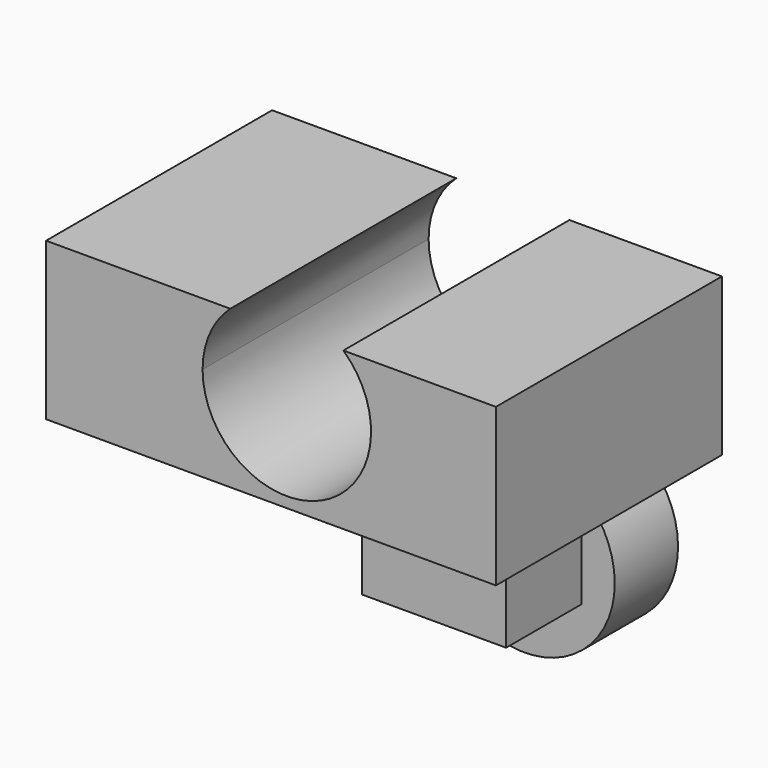
from build123d import *

# Parameters (mm, degrees)
F2_DEPTH = 25
F1_W     = 37.6658551395
F1_H     = 13.7970196083
F3_DEPTH = 25
F4_DEPTH = 25
F6_DEPTH = 300
F7_W     = 21.0016183555
F7_H     = 23.9549651742
F8_ANGLE = 320


with BuildPart() as f2:
    # F0 (on Front) → F2 (new body)
    with BuildSketch(Plane.XZ):
        Polygon((-63.9058277011, 0), (0, 0), (55.5029883981, 0), (55.5029883981, 41.7323634028), (-63.9058277011, 41.7323634028), align=None)
    extrude(amount=F2_DEPTH)

    # F3 (add): a face of the model
    f3_faces = [f2.faces().sort_by_distance(p)[0] for p in [
        (-4.2014196515, -25, 20.8661817014),
    ]]
    extrude(f3_faces, amount=F3_DEPTH)

    # F4 (add): a face of the model
    f4_faces = [f2.faces().sort_by_distance(p)[0] for p in [
        (-4.2014196515, 0, 20.8661817014),
    ]]
    extrude(f4_faces, amount=F4_DEPTH)

    # F5 (on face) → F6 (cut)
    with BuildSketch(Plane(origin=(0, 25, 0), x_dir=(-1, 0, 0), z_dir=(0, 1, 0))):
        with BuildLine():
            Line((-15.0098233938, 41.7323634028), (15.0098233938, 41.7323634028))
            ThreePointArc((15.0098233938, 41.7323634028), (0, 47.5189849051), (-15.0098233938, 41.7323634028))
        make_face()
        with BuildLine():
            ThreePointArc((-15.0098233938, 41.7323634028), (-9.0651881117, 4.7186498209), (22.3601791324, 25.1588057727))
            ThreePointArc((22.3601791324, 25.1588057727), (20.4401559518, 34.2239938844), (15.0098233938, 41.7323634028))
            Line((15.0098233938, 41.7323634028), (-15.0098233938, 41.7323634028))
        make_face()
    extrude(amount=-F6_DEPTH, mode=Mode.SUBTRACT)


with BuildPart() as f2b:
    # F1 (on Front) → F2, piece 2 (new body)
    with BuildSketch(Plane.XZ):
        with Locations((-18.8329275697, -6.8985098042)):
            Rectangle(F1_W, F1_H)
        Polygon((38.217741996, 0), (0, 0), (0, -13.7970196083), (0, -30.3534418344), (38.217741996, -30.3534418344), align=None)
    extrude(amount=F2_DEPTH)


with BuildPart() as f8:
    # F7 (on Right) → F8 (revolve)
    with BuildSketch(Plane.YZ):
        with Locations((39.3780265003, -29.8616662621)):
            Rectangle(F7_W, F7_H)
    revolve(axis=Axis((0, 39.3780265003, -41.8391488492), (0, -1, 0)), revolution_arc=F8_ANGLE)


solid = Compound([f2.part, f2b.part, f8.part])
